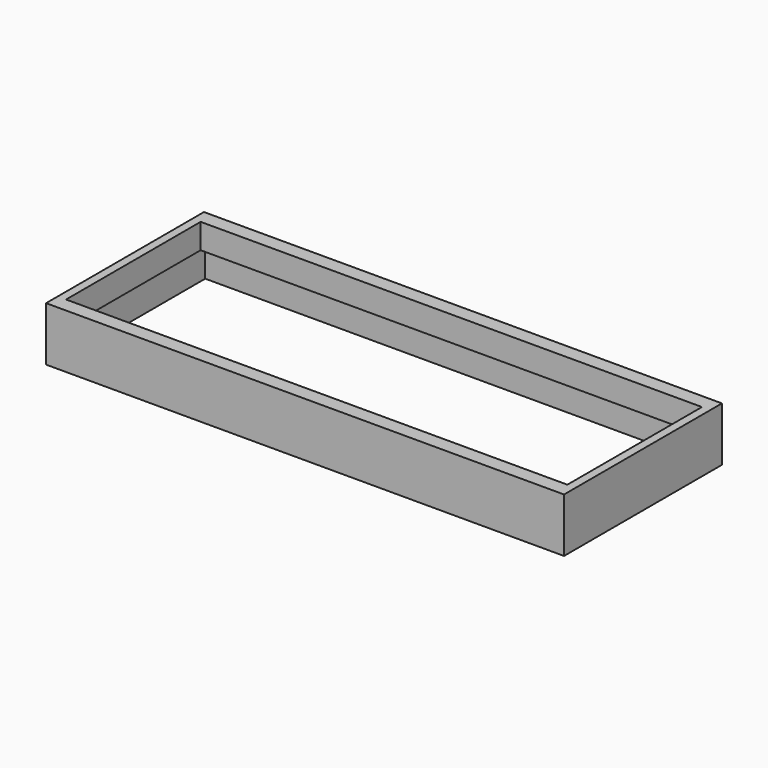
from build123d import *

# Parameters (mm, degrees)
F0_W     = 124.4
F0_H     = 47.4
F0_W_2   = 121.4
F0_H_2   = 44.4
F1_DEPTH = 7
F2_W     = 124.4
F2_H     = 47.4
F2_W_2   = 121.4
F2_H_2   = 44.4
F2_W_3   = 120.4
F2_H_3   = 40.4
F3_DEPTH = 6


with BuildPart() as f1:
    # F0 (on Top) → F1 (new body)
    with BuildSketch(Plane.XY):
        Rectangle(F0_W, F0_H)
        Rectangle(F0_W_2, F0_H_2, mode=Mode.SUBTRACT)
    extrude(amount=F1_DEPTH)

    # F2 (on face) → F3 (join)
    with BuildSketch(Plane.XY.offset(7)):
        Rectangle(F2_W, F2_H)
        Rectangle(F2_W_2, F2_H_2, mode=Mode.SUBTRACT)
        Rectangle(F2_W_2, F2_H_2)
        Rectangle(F2_W_3, F2_H_3, mode=Mode.SUBTRACT)
    extrude(amount=F3_DEPTH)


solid = f1.part
